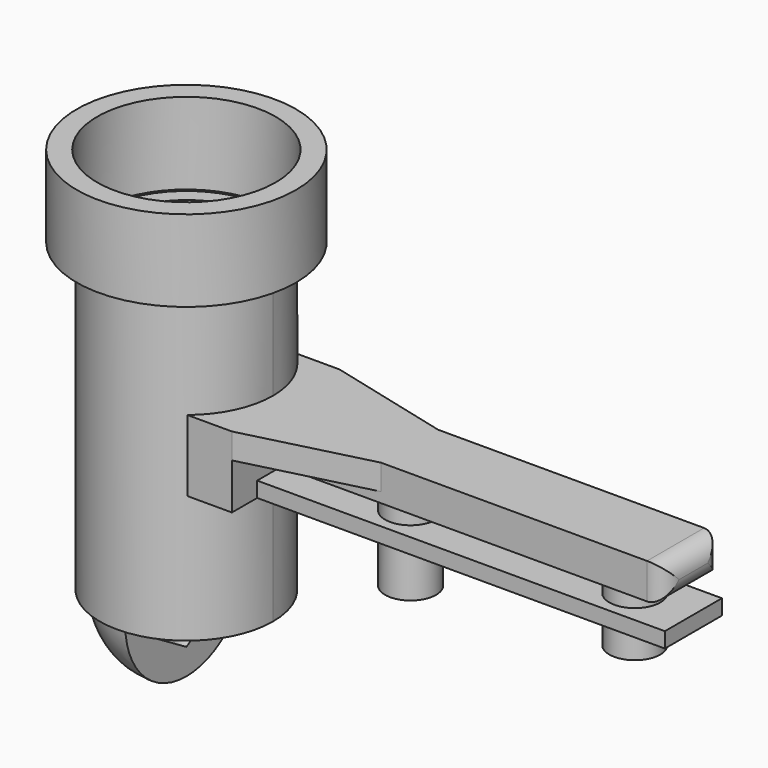
from build123d import *

# Parameters (mm, degrees)
F1_DEPTH  = 7.5
F4_W      = 4.8718336038
F4_H      = 6.594719131
F5_DEPTH  = 1.25
F9_W      = 3.5
F9_H      = 0.75
F10_DEPTH = 20
F14_DEPTH = 20
F15_D     = 2.5
F15_DEPTH = 5
F15_TIP   = 0.7510757738
F16_DEPTH = 5
F17_DEPTH = 1
F18_DEPTH = 4
F20_DEPTH = 1.25
F21_DEPTH = 25
F22_R     = 5.375
F22_R_2   = 4.375
F23_DEPTH = 4
F24_R     = 0.87499
F25_ANGLE = 90
F26_D     = 5.99
F26_DEPTH = 6
F26_TIP   = 1.799577554


# Not quite as in the source:
# - a fillet or chamfer is up to 0.001 mm smaller than in the source, because OpenCascade refuses the exact size
# - a feature names something its author has since deleted; it is built from what else it names


with BuildPart() as f1:
    # F0 (on Top) → F1 (new body, symmetric)
    with BuildSketch(Plane.XY):
        with BuildLine():
            ThreePointArc((0.4, 3.4770677301), (2.6124700955, 2.3291629398), (3.5, 0))
            ThreePointArc((3.5, 0), (2.4748737342, -2.4748737342), (0, -3.5))
            Line((0, -3.5), (0, -4.25))
            ThreePointArc((0, -4.25), (3.00520382, -3.00520382), (4.25, 0))
            ThreePointArc((4.25, 0), (3.1434455618, 2.860288447), (0.4, 4.2311345996))
            Line((0.4, 4.2311345996), (0.4, 3.4770677301))
        make_face()
        with BuildLine():
            Line((0, -4.25), (0, -3.5))
            ThreePointArc((0, -3.5), (-3.5, 0), (0, 3.5))
            Line((0, 3.5), (0, 4.25))
            ThreePointArc((0, 4.25), (-4.25, 0), (0, -4.25))
        make_face()
    extrude(amount=F1_DEPTH, both=True)

    # F4 (on Top) → F5 (join, symmetric)
    with BuildSketch(Plane.XY):
        with Locations((2.4359168019, 0)):
            Rectangle(F4_W, F4_H)
    extrude(amount=F5_DEPTH, both=True)

    # F9 (on offset) → F10 (join)
    with BuildSketch(Plane.YZ.offset(4.8718336038)):
        with Locations((0, 0.875)):
            Rectangle(F9_W, F9_H)
    extrude(amount=F10_DEPTH)

    # F12 (on offset) → F16 (join)
    with BuildSketch(Plane.XY.offset(1.25)):
        with BuildLine():
            Line((12.25, 0), (11, 0))
            Line((11, 0), (9.75, 0))
            ThreePointArc((9.75, 0), (11, -1.25), (12.25, 0))
        make_face()
        with BuildLine():
            Line((9.75, 0), (11, 0))
            Line((11, 0), (12.25, 0))
            ThreePointArc((12.25, 0), (11, 1.25), (9.75, 0))
        make_face()
    extrude(amount=-F16_DEPTH)

    # F17 (add): a face of the model
    f17_faces = [f1.faces().sort_by_distance(p)[0] for p in [
        (13.8735829145, 0, 1.25),
    ]]
    extrude(f17_faces, amount=F17_DEPTH)

    # F12 (on offset) → F18 (join)
    with BuildSketch(Plane.XY.offset(1.25)):
        with BuildLine():
            ThreePointArc((23.25, 0), (22, 1.25), (20.75, 0))
            ThreePointArc((20.75, 0), (22, -1.25), (23.25, 0))
        make_face()
    extrude(amount=-F18_DEPTH)

    # F19 (on face) → F20 (join)
    with BuildSketch(Plane.XY.offset(2.25)):
        Polygon((10.9490072355, 1.75), (4.8718336038, 3.2973595655), (4.8718336038, 1.75), align=None)
        Polygon((4.8718336038, -1.75), (4.8718336038, -3.2973595655), (10.9490072355, -1.75), align=None)
    extrude(amount=-F20_DEPTH)

    # F21 (cut): a face of the model
    f21_faces = [f1.faces().sort_by_distance(p)[0] for p in [
        (1.5030375026, 0, 1.25),
    ]]
    extrude(f21_faces, amount=-F21_DEPTH, mode=Mode.SUBTRACT)

    # F24 (radius 0.875 in the source; OpenCascade refuses exactly that, so slightly less here)
    f24_edges = [f1.edges().sort_by_distance(p)[0] for p in [
        (24.871834, 0, 2.25),
        (24.871834, -1.75, 1.375),
        (24.871834, 0, 0.5),
        (24.871834, 1.75, 1.375),
    ]]
    fillet(f24_edges, radius=F24_R)

    # F3 (on offset) → F25 (revolve)
    with BuildSketch(Plane.XY.offset(-7.5)):
        with BuildLine():
            Line((0, -3.7489147878), (0, 3.7510852122))
            ThreePointArc((0, 3.7510852122), (-3.75, 0.0010852122), (0, -3.7489147878))
        make_face()
    revolve(axis=Axis((0, 0.0010852122, -7.5), (0, -1, 0)), revolution_arc=F25_ANGLE)

    # F26
    with Locations(Plane.XY.offset(-2.18)):
        with Locations((0, 0)):
            Hole(F26_D / 2, depth=F26_DEPTH)
            with Locations((0, 0, -(F26_DEPTH + F26_TIP / 2))):  # 118° drill point
                Cone(0, F26_D / 2, F26_TIP, mode=Mode.SUBTRACT)


with BuildPart() as f14:
    # F9 (on offset) → F14 (new body)
    with BuildSketch(Plane.YZ.offset(4.8718336038)):
        with Locations((0, -0.875)):
            Rectangle(F9_W, F9_H)
    extrude(amount=F14_DEPTH)

    # F15
    with Locations(Plane.XY.offset(1.25)):
        with Locations((11, 0), (22, 0)):
            Hole(F15_D / 2, depth=F15_DEPTH)
            with Locations((0, 0, -(F15_DEPTH + F15_TIP / 2))):  # 118° drill point
                Cone(0, F15_D / 2, F15_TIP, mode=Mode.SUBTRACT)


with BuildPart() as f23:
    # F22 (on face) → F23 (new body)
    with BuildSketch(Plane.XY.offset(7.5)):
        Circle(F22_R)
        Circle(F22_R_2, mode=Mode.SUBTRACT)
    extrude(amount=F23_DEPTH)


solid = Compound([f1.part, f14.part, f23.part])
